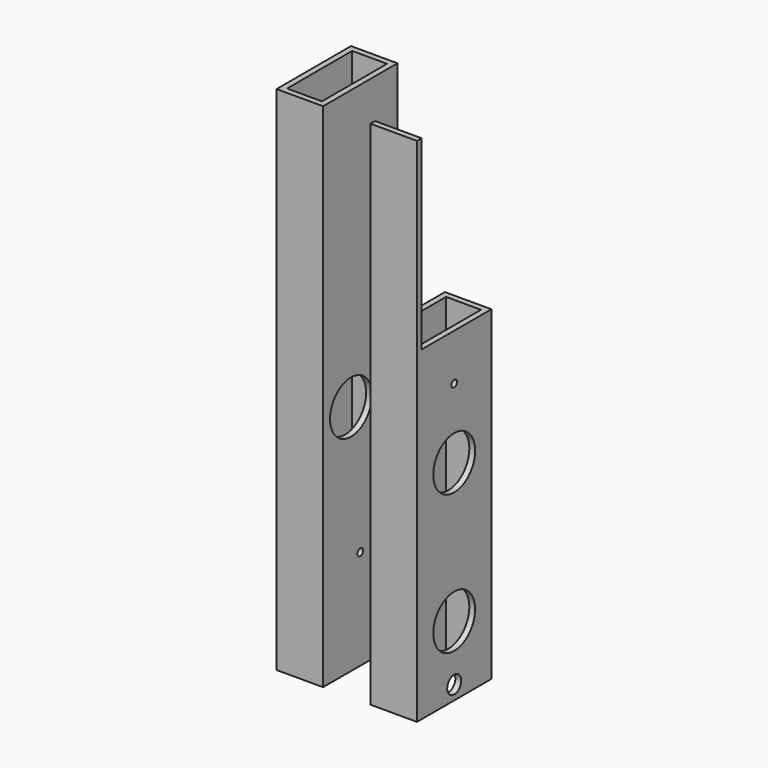
from build123d import *

# Parameters (mm, degrees)
F0_W      = 25.4
F0_H      = 50.8
F0_W_2    = 19.05
F0_H_2    = 44.45
F1_DEPTH  = 177.8
F2_R      = 1.905
F2_R_2    = 14.2875
F2_R_3    = 4.7625
F3_DEPTH  = 25.4
F4_W      = 25.4
F4_H      = 50.8
F4_W_2    = 19.05
F4_H_2    = 44.45
F5_DEPTH  = 279.4
F6_R      = 1.905
F7_DEPTH  = 25.4
F8_R      = 14.2875
F9_DEPTH  = 25.4
F11_DEPTH = 101.6


# Not quite as in the source:
# - a feature names something its author has since deleted; it is built from what else it names


with BuildPart() as f1:
    # F0 (on Top) → F1 (new body)
    with BuildSketch(Plane.XY):
        with Locations((12.7, 25.4)):
            Rectangle(F0_W, F0_H)
        with Locations((12.7, 25.4)):
            Rectangle(F0_W_2, F0_H_2, mode=Mode.SUBTRACT)
    extrude(amount=F1_DEPTH)

    # F2 (on face) → F3 (cut, through all)
    with BuildSketch(Plane.YZ.offset(25.4)):
        with Locations((25.4, 152.4)):
            Circle(F2_R)
        with Locations((25.4, 38.1)):
            Circle(F2_R_2)
        with Locations((25.4, 7.62)):
            Circle(F2_R_3)
        with Locations((25.4, 114.3)):
            Circle(F2_R_2)
    extrude(amount=-F3_DEPTH, mode=Mode.SUBTRACT)

    # F10 (on face) → F11 (join)
    with BuildSketch(Plane.XY.offset(177.8)):
        Polygon((0, 3.175), (0, 0), (25.4, 0), (25.4, 3.175), (22.225, 3.175), (3.175, 3.175), align=None)
    extrude(amount=F11_DEPTH)


with BuildPart() as f5:
    # F4 (on Top) → F5 (new body)
    with BuildSketch(Plane.XY):
        with Locations((-38.6022577927, 25.4)):
            Rectangle(F4_W, F4_H)
        with Locations((-38.6022577927, 25.4)):
            Rectangle(F4_W_2, F4_H_2, mode=Mode.SUBTRACT)
    extrude(amount=F5_DEPTH)

    # F6 (on face) → F7 (cut, through all)
    with BuildSketch(Plane(origin=(-51.3022577927, 0, 0), x_dir=(0, -1, 0), z_dir=(-1, 0, 0))):
        with Locations((-25.4, 54.61)):
            Circle(F6_R)
    extrude(amount=-F7_DEPTH, mode=Mode.SUBTRACT)

    # F8 (on face) → F9 (cut, through all)
    with BuildSketch(Plane(origin=(-51.3022577927, 0, 0), x_dir=(0, -1, 0), z_dir=(-1, 0, 0))):
        with Locations((-19.05, 127)):
            Circle(F8_R)
    extrude(amount=-F9_DEPTH, mode=Mode.SUBTRACT)


solid = Compound([f1.part, f5.part])
